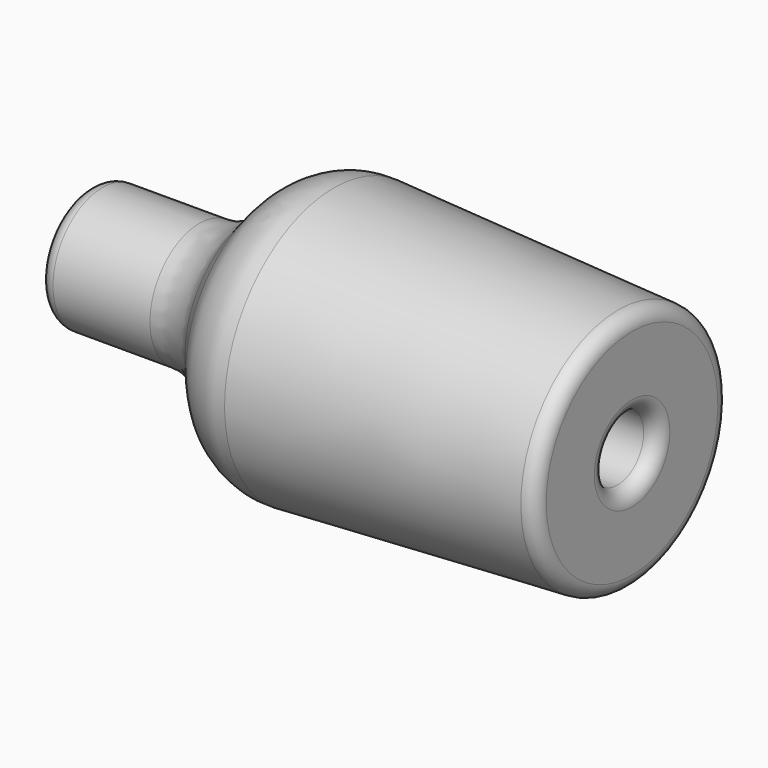
from build123d import *

# Parameters (mm, degrees)
F2_R = 0.99999
F3_R = 5


# Not quite as in the source:
# - a fillet or chamfer is up to 0.001 mm smaller than in the source, because OpenCascade refuses the exact size


with BuildPart() as f1:
    # F0 (on Front) → F1 (revolve)
    with BuildSketch(Plane.XZ):
        Polygon((0, 4.25), (0, 2.25), (14.4355785643, 2.25), (37.4355785643, 2.25), (37.4355785643, 8.3307377657), (14.4355785643, 9.5361166892), (10, 4.25), align=None)
    revolve(axis=Axis((-40, 0, 0), (1, 0, 0)))

    # F2 (radius 1 in the source; OpenCascade refuses exactly that, so slightly less here)
    f2_edges = [f1.edges().sort_by_distance(p)[0] for p in [
        (0, 0, -4.25),
        (37.435579, 0, -8.330738),
        (37.435579, 0, -2.25),
        (0, 0, -2.25),
    ]]
    fillet(f2_edges, radius=F2_R)

    # F3
    f3_edges = [f1.edges().sort_by_distance(p)[0] for p in [
        (14.435579, 0, -9.536117),
        (10, 0, -4.25),
    ]]
    fillet(f3_edges, radius=F3_R)


solid = f1.part
